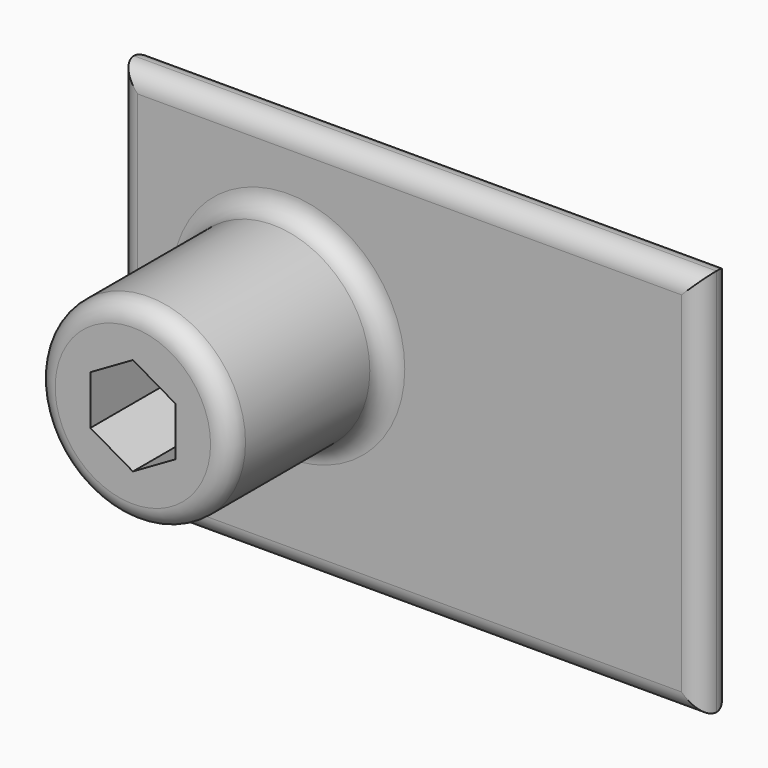
from build123d import *

# Parameters (mm, degrees)
F0_W     = 76.2
F0_H     = 50.8
F1_DEPTH = 5.08
F2_R     = 12.7
F3_DEPTH = 25.4
F5_DEPTH = 12.7
F6_R     = 2.38125
F7_DEPTH = 17.78
F8_R     = 2.53999


# Not quite as in the source:
# - a fillet or chamfer is up to 0.001 mm smaller than in the source, because OpenCascade refuses the exact size


with BuildPart() as f1:
    # F0 (on Front) → F1 (new body)
    with BuildSketch(Plane.XZ):
        Rectangle(F0_W, F0_H)
    extrude(amount=F1_DEPTH)

    # F2 (on face) → F3 (join)
    with BuildSketch(Plane.XZ.offset(5.08)):
        with Locations((-15.875, 2.54)):
            Circle(F2_R)
    extrude(amount=F3_DEPTH)

    # F4 (on face) → F5 (cut)
    with BuildSketch(Plane.XZ.offset(30.48)):
        Polygon((-10.31875, 5.7479024332), (-15.875, 8.9558048664), (-21.43125, 5.7479024332), (-21.43125, -0.6679024332), (-15.875, -3.8758048664), (-10.31875, -0.6679024332), align=None)
    extrude(amount=-F5_DEPTH, mode=Mode.SUBTRACT)

    # F6 (on face) → F7 (cut, through all)
    with BuildSketch(Plane.XZ.offset(17.78)):
        with Locations((-15.875, 2.54)):
            Circle(F6_R)
    extrude(amount=-F7_DEPTH, mode=Mode.SUBTRACT)

    # F8 (radius 2.54 in the source; OpenCascade refuses exactly that, so slightly less here)
    f8_edges = [f1.edges().sort_by_distance(p)[0] for p in [
        (-28.575, -30.48, 2.54),
        (-28.575, -5.08, 2.54),
        (0, -5.08, 25.4),
        (38.1, -5.08, 0),
        (0, -5.08, -25.4),
        (-38.1, -5.08, 0),
        (0, 0, -25.4),
        (-38.1, 0, 0),
        (38.1, 0, 0),
        (0, 0, 25.4),
    ]]
    fillet(f8_edges, radius=F8_R)


solid = f1.part
